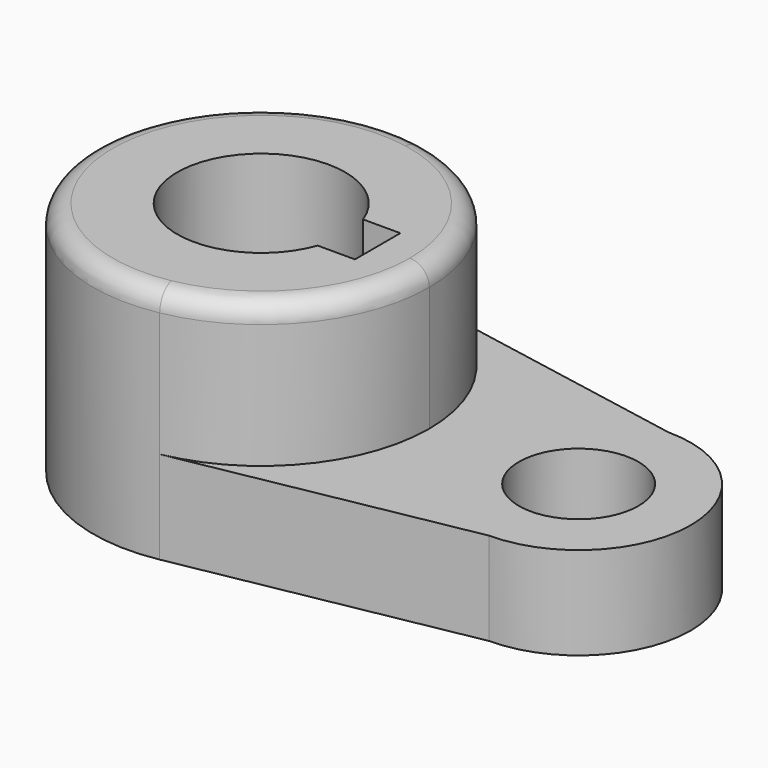
from build123d import *

# Parameters (mm, degrees)
F1_DEPTH = 40.2336
F0_R     = 10.16
F2_DEPTH = 15.7734
F3_R     = 3.302


# Not quite as in the source:
# - a feature names something its author has since deleted; it is built from what else it names


with BuildPart() as f1:
    # F0 (on Top) → F1 (new body)
    with BuildSketch(Plane.XY):
        with BuildLine():
            ThreePointArc((5.2118165727, -28.0956863773), (21.9710978739, -18.2702348977), (28.575, 0))
            ThreePointArc((28.575, 0), (21.9710978739, 18.2702348977), (5.2118165727, 28.0956863773))
            ThreePointArc((5.2118165727, 28.0956863773), (-28.575, 0), (5.2118165727, -28.0956863773))
        make_face()
        with BuildLine():
            ThreePointArc((13.4477648793, -4.826), (-14.2875, 0), (13.4477648793, 4.826))
            Line((13.4477648793, 4.826), (19.7977648793, 4.826))
            Line((19.7977648793, 4.826), (19.7977648793, -4.826))
            Line((19.7977648793, -4.826), (13.4477648793, -4.826))
        make_face(mode=Mode.SUBTRACT)
    extrude(amount=F1_DEPTH)

    # F0 (on Top) → F2 (join)
    with BuildSketch(Plane.XY):
        with BuildLine():
            ThreePointArc((5.2118165727, 28.0956863773), (21.9710978739, 18.2702348977), (28.575, 0))
            ThreePointArc((28.575, 0), (21.9710978739, -18.2702348977), (5.2118165727, -28.0956863773))
            Line((5.2118165727, -28.0956863773), (53.975, -19.05))
            ThreePointArc((53.975, -19.05), (34.925, 0), (53.975, 19.05))
            Line((53.975, 19.05), (5.2118165727, 28.0956863773))
        make_face()
        with BuildLine():
            ThreePointArc((73.025, 0), (67.4453841816, 13.4703841816), (53.975, 19.05))
            ThreePointArc((53.975, 19.05), (34.925, 0), (53.975, -19.05))
            ThreePointArc((53.975, -19.05), (67.4453841816, -13.4703841816), (73.025, 0))
        make_face()
        with Locations((53.975, 0)):
            Circle(F0_R, mode=Mode.SUBTRACT)
    extrude(amount=F2_DEPTH)

    # F3
    f3_edges = [f1.edges().sort_by_distance(p)[0] for p in [
        (-5.211817, 28.095686, 40.2336),
    ]]
    fillet(f3_edges, radius=F3_R)


solid = f1.part
